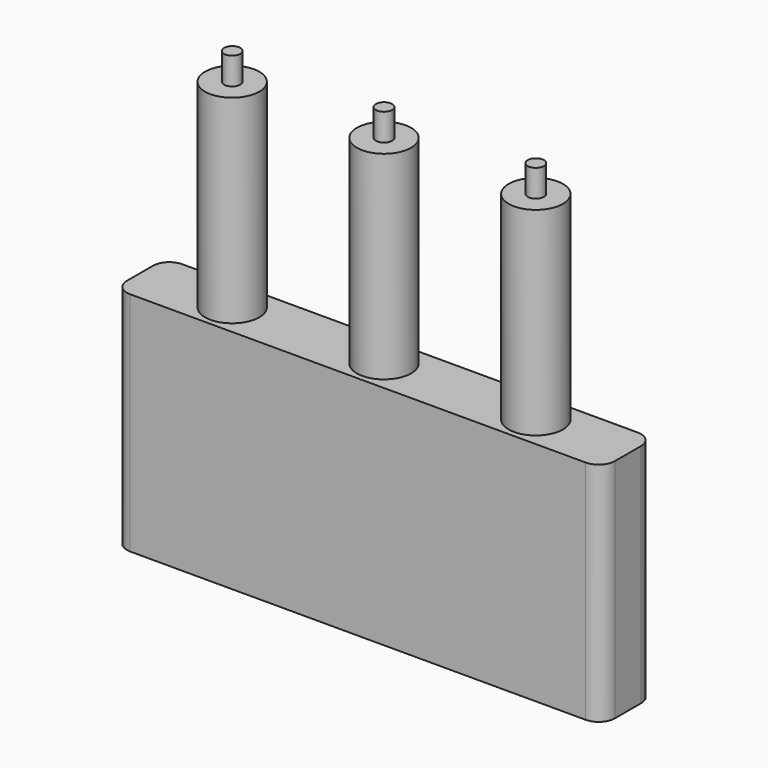
from build123d import *

# Parameters (mm, degrees)
F0_W     = 90
F0_H     = 41.77
F1_DEPTH = 6
F3_DEPTH = 36.63
F4_R     = 3
F5_R     = 1.5
F6_DEPTH = 5


with BuildPart() as f1:
    # F0 (on Front) → F1 (new body, symmetric)
    with BuildSketch(Plane.XZ):
        Rectangle(F0_W, F0_H)
    extrude(amount=F1_DEPTH, both=True)

    # F2 (on face) → F3 (join)
    with BuildSketch(Plane.XY.offset(20.885)):
        with BuildLine():
            Line((-28, 0), (-23, 0))
            ThreePointArc((-23, 0), (-28, 5), (-33, 0))
            Line((-33, 0), (-28, 0))
        make_face()
        with BuildLine():
            ThreePointArc((-33, 0), (-28, -5), (-23, 0))
            Line((-23, 0), (-28, 0))
            Line((-28, 0), (-33, 0))
        make_face()
        with BuildLine():
            Line((-5, 0), (0, 0))
            Line((0, 0), (5, 0))
            ThreePointArc((5, 0), (0, 5), (-5, 0))
        make_face()
        with BuildLine():
            Line((5, 0), (0, 0))
            Line((0, 0), (-5, 0))
            ThreePointArc((-5, 0), (0, -5), (5, 0))
        make_face()
        with BuildLine():
            ThreePointArc((33, 0), (28, 5), (23, 0))
            ThreePointArc((23, 0), (28, -5), (33, 0))
        make_face()
    extrude(amount=F3_DEPTH)

    # F4
    f4_edges = [f1.edges().sort_by_distance(p)[0] for p in [
        (45, -6, 0),
        (45, 6, 0),
        (-45, -6, 0),
        (-45, 6, 0),
    ]]
    fillet(f4_edges, radius=F4_R)

    # F5 (on face) → F6 (join)
    with BuildSketch(Plane.XY.offset(57.515)):
        with Locations((-28, 0)):
            Circle(F5_R)
        Circle(F5_R)
        with Locations((28, 0)):
            Circle(F5_R)
    extrude(amount=F6_DEPTH)


solid = f1.part
